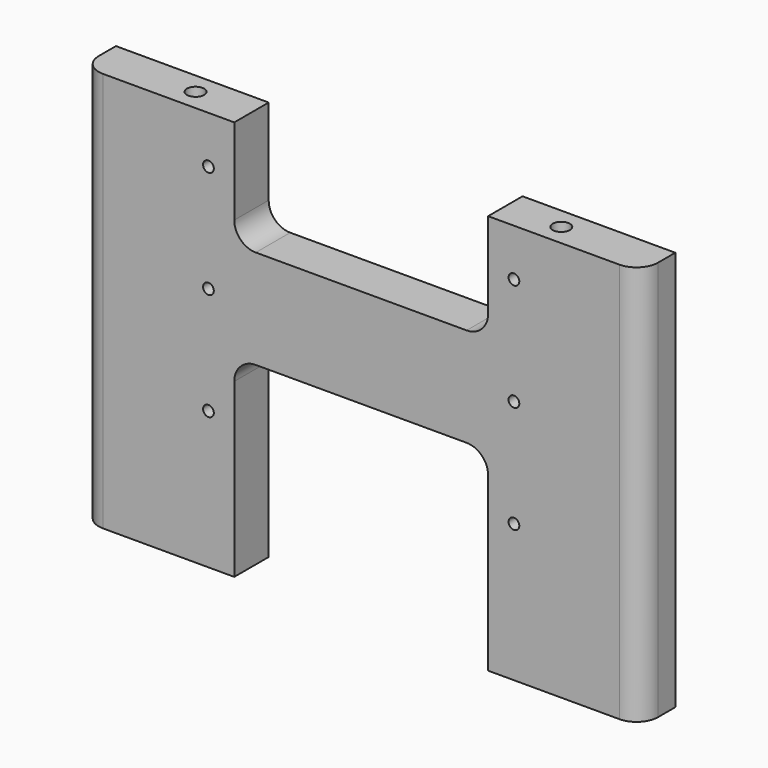
from build123d import *

# Parameters (mm, degrees)
F0_R           = 1.25
F1_DEPTH       = 10
F2_R           = 5
F5_D           = 4
F5_DEPTH       = 15
F5_TIP         = 1.2017212381
F5_ON_F4_D     = 4
F5_ON_F4_DEPTH = 15
F5_ON_F4_TIP   = 1.2017212381


with BuildPart() as f1:
    # F0 (on Front) → F1 (new body)
    with BuildSketch(Plane.XZ):
        Polygon((-65, 43.3330013267), (-65, -49.6669986733), (-29.5, -49.6669986733), (-29.5, -4.6669986733), (0, -4.6669986733), (0, 18.3330013267), (-29.5, 18.3330013267), (-29.5, 43.3330013267), align=None)
        with Locations((-35.5, -42.6669986733)):
            Circle(F0_R, mode=Mode.SUBTRACT)
        with Locations((-35.5, -17.6669986733)):
            Circle(F0_R, mode=Mode.SUBTRACT)
        with Locations((-35.5, 7.3330013267)):
            Circle(F0_R, mode=Mode.SUBTRACT)
        with Locations((-35.5, 32.3330013267)):
            Circle(F0_R, mode=Mode.SUBTRACT)
        with Locations((-35.5, -42.6669986733)):
            Circle(F0_R)
    extrude(amount=F1_DEPTH)

    # F2
    f2_edges = [f1.edges().sort_by_distance(p)[0] for p in [
        (-65, -10, -3.166999),
        (-29.5, -5, -4.666999),
        (-29.5, -5, 18.333001),
    ]]
    fillet(f2_edges, radius=F2_R)

    # F5
    with Locations(Plane.XY.offset(43.3330013267)):
        with Locations((-42.5, -5)):
            Hole(F5_D / 2, depth=F5_DEPTH)
            with Locations((0, 0, -(F5_DEPTH + F5_TIP / 2))):  # 118° drill point
                Cone(0, F5_D / 2, F5_TIP, mode=Mode.SUBTRACT)

    # F5 on F4
    with Locations(Plane(origin=(0, 0, -49.6669986733), x_dir=(1, 0, 0), z_dir=(0, 0, -1))):
        with Locations((-42.5, 5)):
            Hole(F5_ON_F4_D / 2, depth=F5_ON_F4_DEPTH)
            with Locations((0, 0, -(F5_ON_F4_DEPTH + F5_ON_F4_TIP / 2))):  # 118° drill point
                Cone(0, F5_ON_F4_D / 2, F5_ON_F4_TIP, mode=Mode.SUBTRACT)

    # F6: F1 across plane


with BuildPart() as f1_1:
    add(f1.part)
    add(f1.part.mirror(Plane.YZ))


solid = f1_1.part
